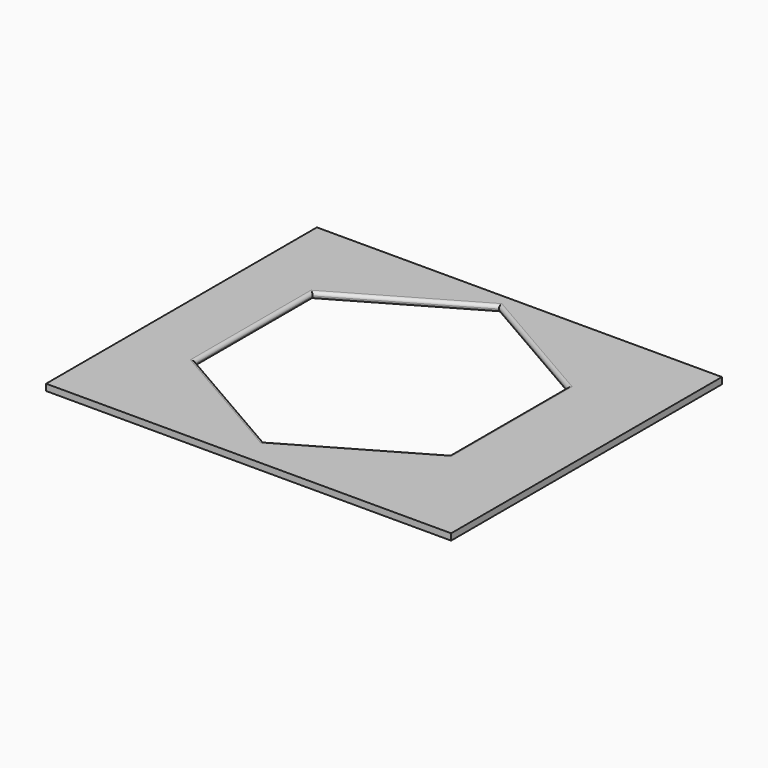
from build123d import *

# Parameters (mm, degrees)
F0_W     = 125.1782737672
F0_H     = 104.6107336879
F1_DEPTH = 2
F2_R     = 0.99999
F3_R     = 0.99999
F4_R     = 0.99999
F5_R     = 0.99999
F6_R     = 0.99999
F7_R     = 0.9999


# Not quite as in the source:
# - a fillet or chamfer is up to 0.001 mm smaller than in the source, because OpenCascade refuses the exact size


with BuildPart() as f1:
    # F0 (on Top) → F1 (new body)
    with BuildSketch(Plane.XY):
        with Locations((2.8369072825, -2.482291311)):
            Rectangle(F0_W, F0_H)
        Polygon((39.3484285011, 22.7178257873), (39.3484285011, -22.7178257873), (0, -45.4356515746), (-39.3484285011, -22.7178257873), (-39.3484285011, 22.7178257873), (0, 45.4356515746), align=None, mode=Mode.SUBTRACT)
    extrude(amount=F1_DEPTH)

    # F2 (radius 1 in the source; OpenCascade refuses exactly that, so slightly less here)
    f2_edges = [f1.edges().sort_by_distance(p)[0] for p in [
        (-19.674214, -34.076739, 2),
        (-19.674214, -34.076739, 0),
    ]]
    fillet(f2_edges, radius=F2_R)

    # F3 (radius 1 in the source; OpenCascade refuses exactly that, so slightly less here)
    f3_edges = [f1.edges().sort_by_distance(p)[0] for p in [
        (-39.348429, 0, 2),
        (-39.348429, 0, 0),
    ]]
    fillet(f3_edges, radius=F3_R)

    # F4 (radius 1 in the source; OpenCascade refuses exactly that, so slightly less here)
    f4_edges = [f1.edges().sort_by_distance(p)[0] for p in [
        (19.674214, -34.076739, 2),
        (19.674214, -34.076739, 0),
    ]]
    fillet(f4_edges, radius=F4_R)

    # F5 (radius 1 in the source; OpenCascade refuses exactly that, so slightly less here)
    f5_edges = [f1.edges().sort_by_distance(p)[0] for p in [
        (39.348429, 0, 2),
        (39.348429, 0, 0),
    ]]
    fillet(f5_edges, radius=F5_R)

    # F6 (radius 1 in the source; OpenCascade refuses exactly that, so slightly less here)
    f6_edges = [f1.edges().sort_by_distance(p)[0] for p in [
        (-19.674214, 34.076739, 2),
        (-19.674214, 34.076739, 0),
    ]]
    fillet(f6_edges, radius=F6_R)

    # F7 (radius 1 in the source; OpenCascade refuses exactly that, so slightly less here)
    f7_edges = [f1.edges().sort_by_distance(p)[0] for p in [
        (19.674214, 34.076739, 2),
        (19.674214, 34.076739, 0),
    ]]
    fillet(f7_edges, radius=F7_R)


solid = f1.part
